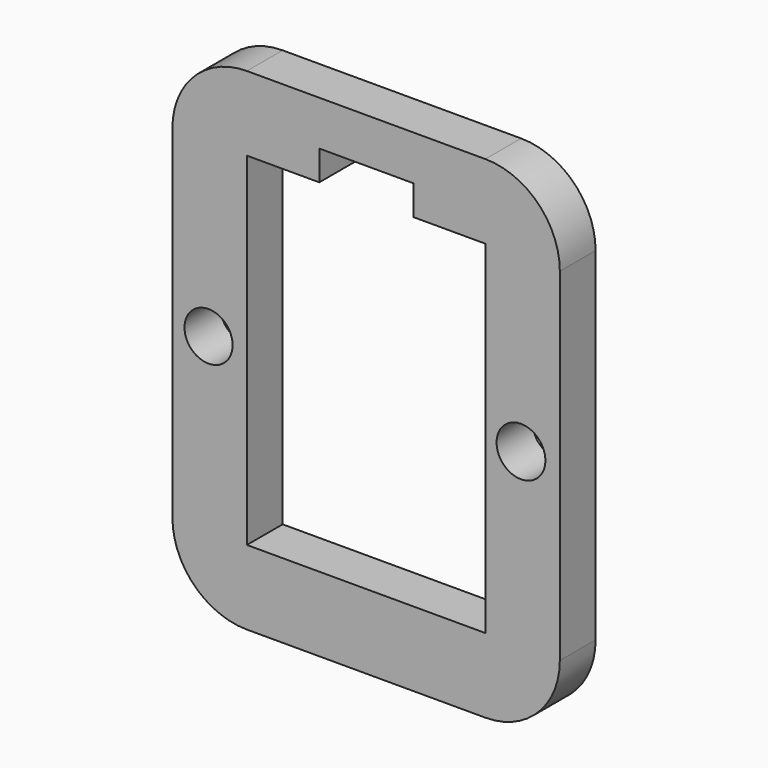
from build123d import *

# Parameters (mm, degrees)
F0_R     = 1.6143877839
F0_R_2   = 1.6384664926
F1_DEPTH = 3


# Not quite as in the source:
# - a feature names something its author has since deleted; it is built from what else it names


with BuildPart() as f1:
    # F0 (on Front) → F1 (new body)
    with BuildSketch(Plane.XZ):
        with BuildLine():
            Line((-39.6336754784, 28), (-39.6336754784, 5))
            ThreePointArc((-39.6336754784, 5), (-38.1692093843, 1.4644660941), (-34.6336754784, 0))
            Line((-34.6336754784, 0), (-18.6336754784, 0))
            ThreePointArc((-18.6336754784, 0), (-15.0981415725, 1.4644660941), (-13.6336754784, 5))
            Line((-13.6336754784, 5), (-13.6336754784, 28))
            ThreePointArc((-13.6336754784, 28), (-15.0981415725, 31.5355339059), (-18.6336754784, 33))
            Line((-18.6336754784, 33), (-34.6336754784, 33))
            ThreePointArc((-34.6336754784, 33), (-38.1692093843, 31.5355339059), (-39.6336754784, 28))
        make_face()
        with Locations((-37.207160145, 16.4869632572)):
            Circle(F0_R, mode=Mode.SUBTRACT)
        Polygon((-34.6336754784, 5), (-34.6336754784, 16.5), (-34.6336754784, 28), (-29.7759659588, 28), (-29.7759659588, 30), (-23.4435740858, 30), (-23.4435740858, 28), (-18.6336754784, 28), (-18.6336754784, 5), align=None, mode=Mode.SUBTRACT)
        with Locations((-16.2413809448, 16.5)):
            Circle(F0_R_2, mode=Mode.SUBTRACT)
    extrude(amount=F1_DEPTH)


solid = f1.part
